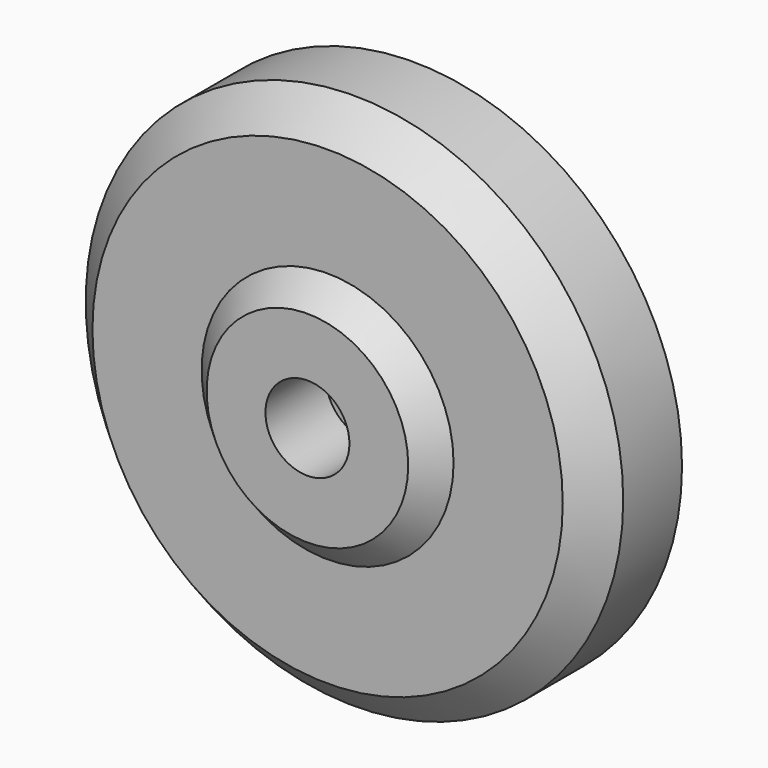
from build123d import *

# Parameters (mm, degrees)
F0_R      = 64
F1_DEPTH  = 25.5
F2_R      = 58
F3_DEPTH  = 1
F4_SIZE   = 8
F5_R      = 30
F6_DEPTH  = 6
F7_SIZE   = 5.99999
F9_R      = 10
F10_DEPTH = 18


# Not quite as in the source:
# - a fillet or chamfer is up to 0.001 mm smaller than in the source, because OpenCascade refuses the exact size


with BuildPart() as f1:
    # F0 (on Front) → F1 (new body)
    with BuildSketch(Plane.XZ):
        Circle(F0_R)
    extrude(amount=F1_DEPTH)

    # F2 (on face) → F3 (cut)
    with BuildSketch(Plane(origin=(0, 0, 0), x_dir=(-1, 0, 0), z_dir=(0, 1, 0))):
        Circle(F2_R)
    extrude(amount=-F3_DEPTH, mode=Mode.SUBTRACT)

    # F4
    f4_edges = [f1.edges().sort_by_distance(p)[0] for p in [
        (-64, -25.5, 0),
    ]]
    chamfer(f4_edges, length=F4_SIZE)

    # F5 (on face) → F6 (join)
    with BuildSketch(Plane.XZ.offset(25.5)):
        Circle(F5_R)
    extrude(amount=F6_DEPTH)

    # F7 (size 6 in the source; OpenCascade refuses exactly that, so slightly less here)
    f7_edges = [f1.edges().sort_by_distance(p)[0] for p in [
        (-30, -31.5, 0),
    ]]
    chamfer(f7_edges, length=F7_SIZE)

    # F9 (on face) → F10 (cut)
    with BuildSketch(Plane.XZ.offset(31.5)):
        Circle(F9_R)
    extrude(amount=-F10_DEPTH, mode=Mode.SUBTRACT)


solid = f1.part
